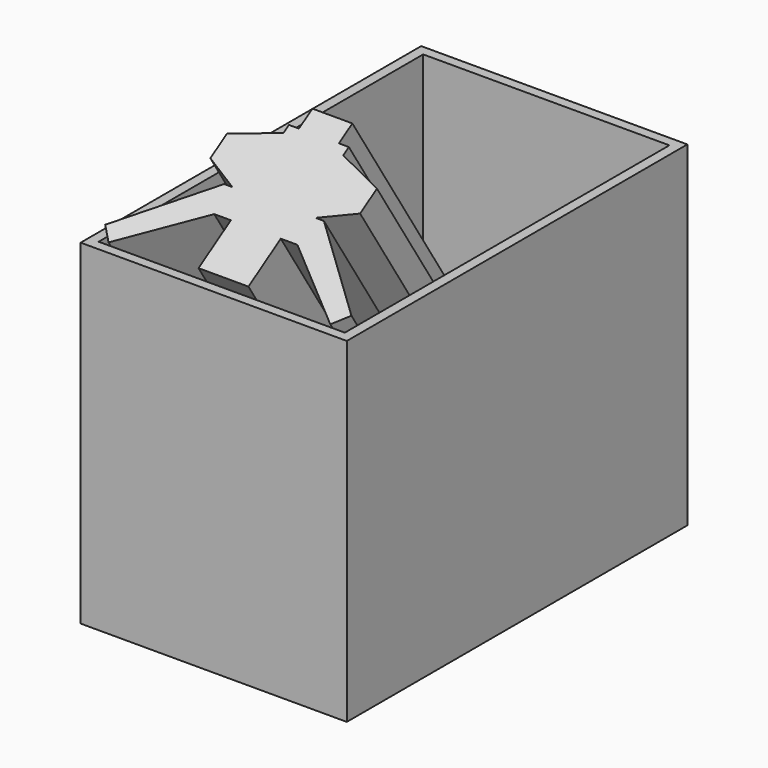
from build123d import *

# Parameters (mm, degrees)
F0_W     = 31.995
F0_H     = 51.168
F1_DEPTH = 20.158
F3_T     = -1.2
F5_REACH = 97.2809453654


with BuildPart() as f1:
    # F0 (on Top) → F1 (new body, symmetric)
    with BuildSketch(Plane.XY):
        Rectangle(F0_W, F0_H)
    extrude(amount=F1_DEPTH, both=True)

    # F3
    f3_openings = [f1.faces().sort_by_distance(p)[0] for p in [
        (0, 0, 20.158),
    ]]
    offset(amount=F3_T, openings=f3_openings)


with BuildPart() as f5:
    f5_end = Plane.XY.offset(-18.958)
    # F4 (on face) → F5 (new body, up to a plane its end follows)
    with BuildSketch(Plane(origin=(0, -16.5150093929, 25.9333592132), x_dir=(1, 0, 0), z_dir=(0, -0.5371524006, 0.8434852094))):
        Polygon((3, -3.2555523465), (5, -3.2555523465), (13.3302325572, -9.7396252559), (14.7975749325, -8.1533091782), (6, -0.0155523465), (5, -0.0155523465), (9, 1.9844476535), (9, 4.9844476535), (3.6, 6.9844476535), (3.6, 7.9844476535), (2.4, 7.9844476535), (2.4, 10.3844476535), (0, 10.3844476535), (-2.4, 10.3844476535), (-2.4, 7.9844476535), (-3.6, 7.9844476535), (-3.6, 6.9844476535), (-9, 4.9844476535), (-9, 1.9844476535), (-5, -0.0155523465), (-6, -0.0155523465), (-14.7975749325, -8.1533091782), (-13.3302325572, -9.7396252559), (-5, -3.2555523465), (-3, -3.2555523465), (-3, -9.0155523465), (0, -9.0155523465), (3, -9.0155523465), align=None)
    f5_long = extrude(amount=-F5_REACH, mode=Mode.PRIVATE)
    add(split(f5_long, bisect_by=f5_end, keep=Keep.TOP, mode=Mode.PRIVATE))


solid = Compound([f1.part, f5.part])
